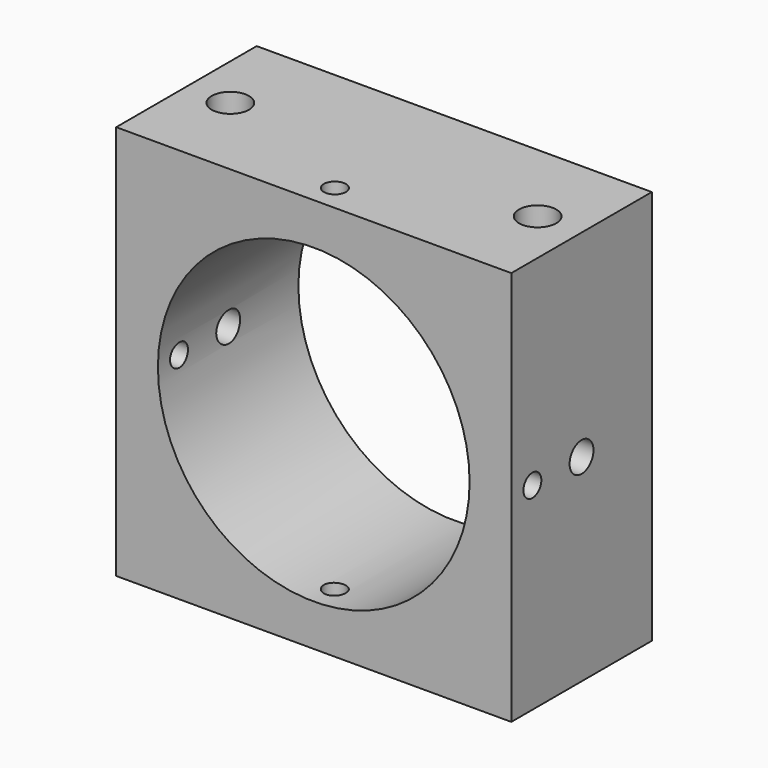
from build123d import *

# Parameters (mm, degrees)
F0_W      = 90
F0_H      = 90
F1_DEPTH  = 40
F3_D      = 71
F5_D      = 5.1054
F6_D      = 6.8
F8_D      = 5
F10_D     = 8.5
F10_DEPTH = 19
F10_TIP   = 2.5536576309


# Not quite as in the source:
# - a feature names something its author has since deleted; it is built from what else it names


with BuildPart() as f1:
    # F0 (on Front) → F1 (new body)
    with BuildSketch(Plane.XZ):
        with Locations((45, 45)):
            Rectangle(F0_W, F0_H)
    extrude(amount=F1_DEPTH)

    # F3 (through all)
    with Locations(Plane.XZ.offset(40)):
        with Locations((45, 45)):
            Hole(F3_D / 2)

    # F5 (through all)
    with Locations(Plane.YZ.offset(90)):
        with Locations((-34, 45)):
            Hole(F5_D / 2)

    # F6 (through all)
    with Locations(Plane.YZ.offset(90)):
        with Locations((-20, 45)):
            Hole(F6_D / 2)

    # F8 (through all)
    with Locations(Plane.XY.offset(90)):
        with Locations((45, -34)):
            Hole(F8_D / 2)

    # F10
    with Locations(Plane.XY.offset(90)):
        with Locations((10, -20), (80, -20)):
            Hole(F10_D / 2, depth=F10_DEPTH)
            with Locations((0, 0, -(F10_DEPTH + F10_TIP / 2))):  # 118° drill point
                Cone(0, F10_D / 2, F10_TIP, mode=Mode.SUBTRACT)


solid = f1.part
